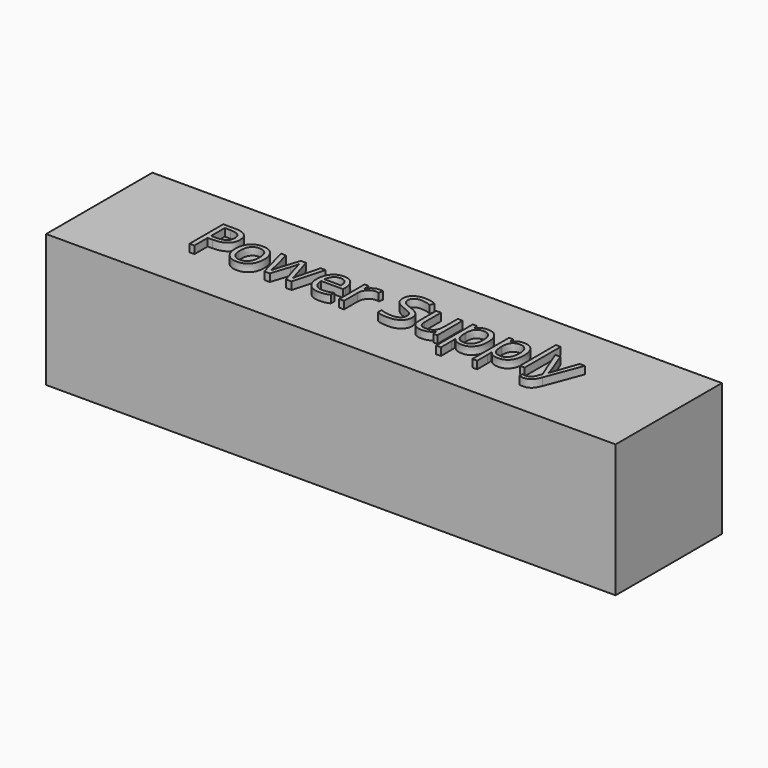
from build123d import *

# Parameters (mm, degrees)
F0_W         = 150
F0_H         = 35
F1_DEPTH     = 35
F3_TEXT_SIZE = 15.5710184419
F4_DEPTH     = 2


# Not quite as in the source:
# - Text() gives the source's letters only with a copy of the font that has no kerning and outlines rounded to 1/6400 em; it was checked with that copy


with BuildPart() as f1:
    # F0 (on Top) → F1 (new body)
    with BuildSketch(Plane.XY):
        Rectangle(F0_W, F0_H)
    extrude(amount=F1_DEPTH)

    # F3 (on offset) → F4 (join)
    with BuildSketch(Plane.XY.offset(35)):
        with Locations((-48.3962639726, -5.4498565588)):
            Text('Power Supply', F3_TEXT_SIZE, font='Open Sans', text_align=(TextAlign.LEFT, TextAlign.BOTTOM))
    extrude(amount=F4_DEPTH)


solid = f1.part
